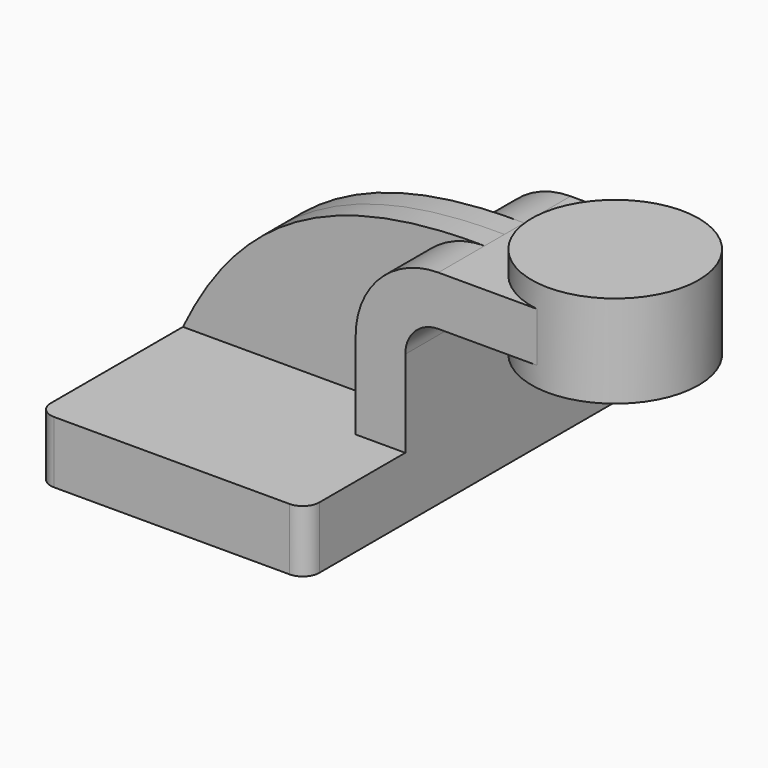
from build123d import *

# Parameters (mm, degrees)
F1_DEPTH = 63.5
F0_W     = 25.1418616311
F0_H     = 15.24
F2_DEPTH = 25.4
F3_DEPTH = 7.62
F5_R     = 5.08
F6_R     = 5.08
F7_R     = 5.08
F8_R     = 5.08


with BuildPart() as f1:
    # F0 (on Front) → F1 (new body, symmetric)
    with BuildSketch(Plane.XZ):
        Polygon((-41.275, -9.525), (41.275, -9.525), (41.275, 9.525), (26.035, 9.525), (-41.275, 9.525), align=None)
    extrude(amount=F1_DEPTH, both=True)

    # F0 (on Front) → F2 (join, symmetric)
    with BuildSketch(Plane.XZ):
        with BuildLine():
            Line((26.035, 9.525), (41.275, 9.525))
            Line((41.275, 9.525), (41.275, 36.195))
            ThreePointArc((41.275, 36.195), (44.2507951031, 43.3792048969), (51.435, 46.355))
            Line((51.435, 46.355), (60.325, 46.355))
            Line((60.325, 46.355), (60.325, 61.595))
            Line((60.325, 61.595), (51.435, 61.595))
            ThreePointArc((51.435, 61.595), (33.4744877579, 54.1555122421), (26.035, 36.195))
            Line((26.035, 36.195), (26.035, 9.525))
        make_face()
        with Locations((72.8959308155, 53.975)):
            Rectangle(F0_W, F0_H)
    extrude(amount=F2_DEPTH, both=True)

    # F0 (on Front) → F3 (join, symmetric)
    with BuildSketch(Plane.XZ):
        with BuildLine():
            add(Edge.make_bspline(
                [(-41.275, 9.525), (-24.5270843474, 44.4972960267), (2.2869093497, 62.1685317942), (51.435, 61.595)],
                knots=[0, 0, 0, 0, 106.3316932998, 106.3316932998, 106.3316932998, 106.3316932998], degree=3))
            Line((-41.275, 9.525), (26.035, 9.525))
            Line((26.035, 9.525), (26.035, 36.195))
            ThreePointArc((26.035, 36.195), (33.4744877579, 54.1555122421), (51.435, 61.595))
        make_face()
    extrude(amount=F3_DEPTH, both=True)

    # F0 (on Front) → F4 (revolve)
    with BuildSketch(Plane.XZ):
        Polygon((85.4668616311, 68.6612712564), (85.4668616311, 61.595), (85.4668616311, 46.355), (85.4668616311, 40.2132712564), (111.125, 40.2132712564), (111.125, 68.6612712564), align=None)
    revolve(axis=Axis((85.4668616311, 0, 57.5081356282), (0, 0, 1)))

    # F5
    f5_edges = [f1.edges().sort_by_distance(p)[0] for p in [
        (41.275, -63.5, 0),
    ]]
    fillet(f5_edges, radius=F5_R)

    # F6
    f6_edges = [f1.edges().sort_by_distance(p)[0] for p in [
        (-41.275, -63.5, 0),
    ]]
    fillet(f6_edges, radius=F6_R)

    # F7
    f7_edges = [f1.edges().sort_by_distance(p)[0] for p in [
        (41.275, 63.5, 0),
    ]]
    fillet(f7_edges, radius=F7_R)

    # F8
    f8_edges = [f1.edges().sort_by_distance(p)[0] for p in [
        (-41.275, 63.5, 0),
    ]]
    fillet(f8_edges, radius=F8_R)


solid = f1.part
